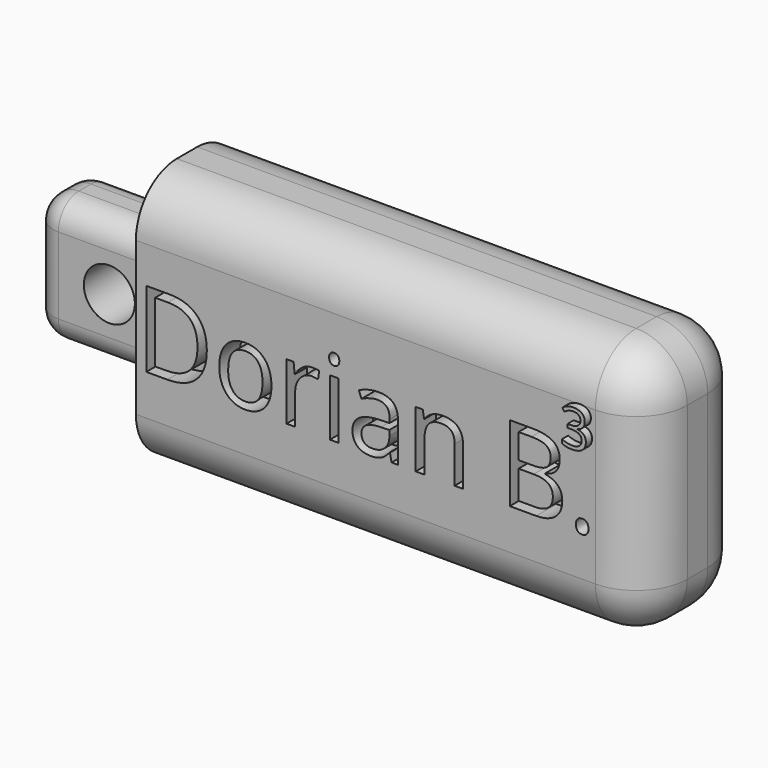
from build123d import *

# Parameters (mm, degrees)
F0_W          = 50.8
F0_H          = 25.4
F1_DEPTH      = 12.7
F2_R          = 5.08
F3_W          = 6.604
F3_H          = 12.7
F4_DEPTH      = 12.7
F5_R          = 2.54
F7_D          = 5.08
F8_TEXT_SIZE  = 10.561940514
F9_DEPTH      = 2.54
F10_TEXT_SIZE = 5.0727305934
F11_DEPTH     = 0.762


# Not quite as in the source:
# - Text() gives the source's letters only with a copy of the font that has no kerning and outlines rounded to 1/6400 em; it was checked with that copy


with BuildPart() as f1:
    # F0 (on Front) → F1 (new body)
    with BuildSketch(Plane.XZ):
        with Locations((25.4, -12.7)):
            Rectangle(F0_W, F0_H)
    extrude(amount=F1_DEPTH)

    # F2
    f2_edges = [f1.edges().sort_by_distance(p)[0] for p in [
        (25.4, -12.7, 0),
        (25.4, 0, 0),
        (50.8, -6.35, 0),
        (50.8, 0, -12.7),
        (50.8, -6.35, -25.4),
        (50.8, -12.7, -12.7),
        (25.4, 0, -25.4),
        (25.4, -12.7, -25.4),
    ]]
    fillet(f2_edges, radius=F2_R)

    # F3 (on face) → F4 (join)
    with BuildSketch(Plane(origin=(0, 0, 0), x_dir=(0, -1, 0), z_dir=(-1, 0, 0))):
        with Locations((6.35, -12.7)):
            Rectangle(F3_W, F3_H)
    extrude(amount=F4_DEPTH)

    # F5
    f5_edges = [f1.edges().sort_by_distance(p)[0] for p in [
        (-6.35, -3.048, -6.35),
        (-6.35, -3.048, -19.05),
        (-6.35, -9.652, -19.05),
        (-6.35, -9.652, -6.35),
        (-12.7, -9.652, -12.7),
        (-12.7, -3.048, -12.7),
        (-12.7, -6.35, -19.05),
        (-12.7, -6.35, -6.35),
    ]]
    fillet(f5_edges, radius=F5_R)

    # F7 (through all)
    with Locations(Plane.XZ.offset(9.652)):
        with Locations((-5.08, -12.7)):
            Hole(F7_D / 2)

    # F8 (on face) → F9 (cut)
    with BuildSketch(Plane.XZ.offset(12.7)):
        with Locations((0, -16.2726013723)):
            Text('Dorian B.', F8_TEXT_SIZE, font='Open Sans', text_align=(TextAlign.LEFT, TextAlign.BOTTOM))
    extrude(amount=-F9_DEPTH, mode=Mode.SUBTRACT)

    # F10 (on face) → F11 (join)
    with BuildSketch(Plane.XZ.offset(12.7)):
        with Locations((42.7816212177, -8.7323660272)):
            Text('3', F10_TEXT_SIZE, font='Open Sans', text_align=(TextAlign.LEFT, TextAlign.BOTTOM))
    extrude(amount=F11_DEPTH)


solid = f1.part
